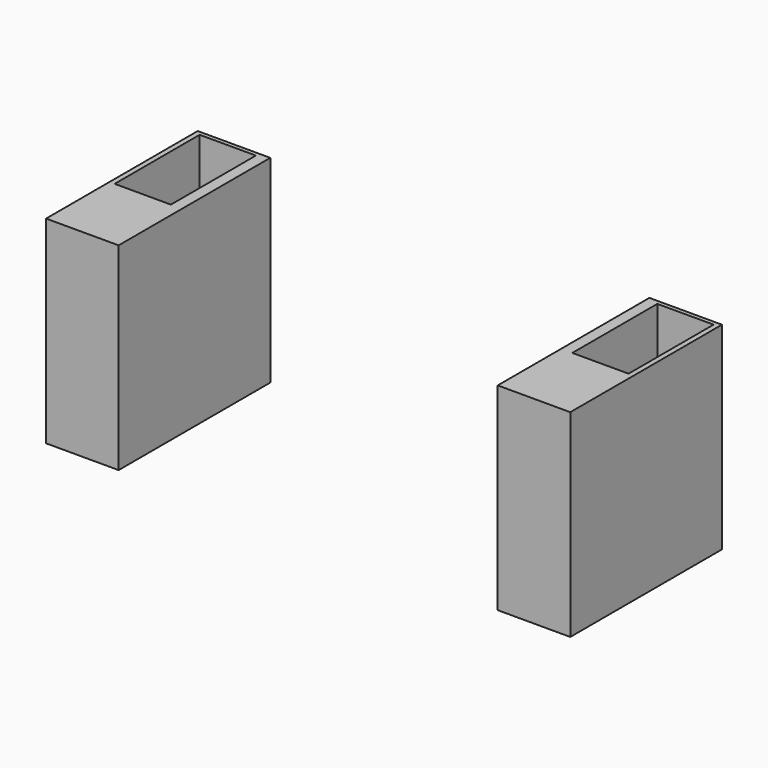
from build123d import *

# Parameters (mm, degrees)
F0_W     = 17.4134043045
F0_H     = 45.5
F0_W_2   = 13.5
F0_H_2   = 25.5
F1_DEPTH = 47.5


# Not quite as in the source:
# - a feature of the source that left no trace in its solid (it failed there, or was rolled back) is left out


with BuildPart() as f1:
    # F0 (on Top) → F1 (new body)
    with BuildSketch(Plane.XY):
        with Locations((104.1058783736, -6.8849609196)):
            Rectangle(F0_W, F0_H)
        with Locations((104.8302046406, 2.1450929129)):
            Rectangle(F0_W_2, F0_H_2, mode=Mode.SUBTRACT)
    extrude(amount=F1_DEPTH)


with BuildPart() as f1b:
    # F0 (on Top) → F1, piece 2 (new body)
    with BuildSketch(Plane.XY):
        with Locations((-4.3075259309, -6.8849609196)):
            Rectangle(F0_W, F0_H)
        with Locations((-5.0318521979, 2.1450929129)):
            Rectangle(F0_W_2, F0_H_2, mode=Mode.SUBTRACT)
    extrude(amount=F1_DEPTH)


solid = Compound([f1.part, f1b.part])
